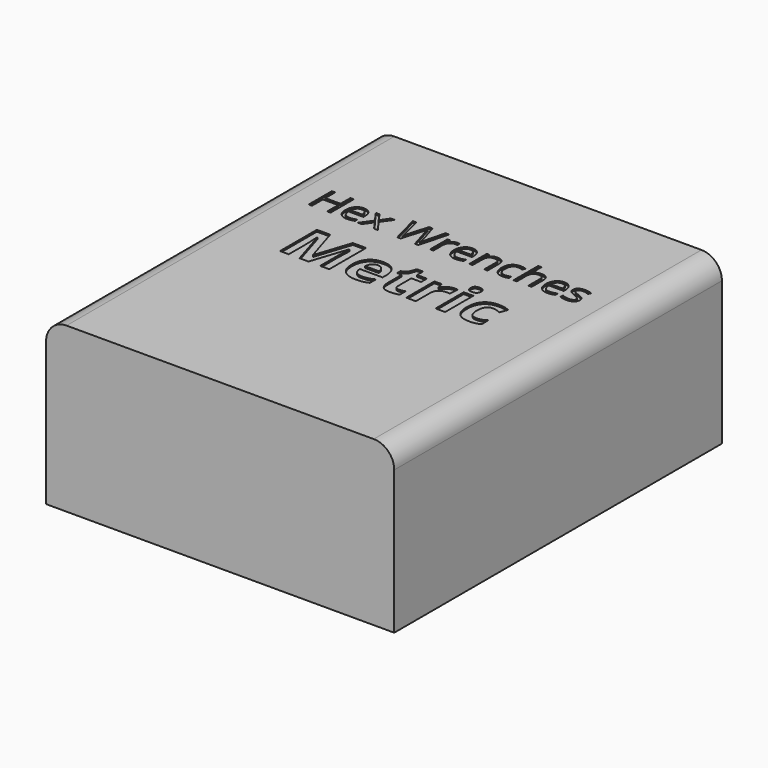
from build123d import *

# Parameters (mm, degrees)
F0_W           = 51.0000002086
F0_H           = 24.0000002086
F0_W_2         = 47
F0_H_2         = 20
F1_DEPTH       = 60
F2_R           = 3
F3_W           = 47
F3_H           = 20
F4_DEPTH       = 1
F5_TEXT_SIZE   = 5.9360942355
F5_TEXT_SIZE_2 = 9.4527740859
F6_DEPTH       = 0.25


# Not quite as in the source:
# - Text() gives the source's letters only with a copy of the font that has no kerning and outlines rounded to 1/6400 em; it was checked with that copy


with BuildPart() as f1:
    # F0 (on Front) → F1 (new body)
    with BuildSketch(Plane.XZ):
        Rectangle(F0_W, F0_H)
        Rectangle(F0_W_2, F0_H_2, mode=Mode.SUBTRACT)
    extrude(amount=F1_DEPTH)

    # F2
    f2_edges = [f1.edges().sort_by_distance(p)[0] for p in [
        (-25.5, -30, 12),
        (25.5, -30, 12),
    ]]
    fillet(f2_edges, radius=F2_R)

    # F3 (on face) → F4 (join)
    with BuildSketch(Plane.XZ.offset(60)):
        Rectangle(F3_W, F3_H)
    extrude(amount=-F4_DEPTH)

    # F5 (on face) → F6 (cut, symmetric)
    with BuildSketch(Plane.XY.offset(12.0000001043)):
        with Locations((-20.1936398028, -19.2833579477)):
            Text('Hex Wrenches', F5_TEXT_SIZE, font='Open Sans', text_align=(TextAlign.LEFT, TextAlign.BOTTOM))
        with Locations((-15.8186899498, -30.32877855)):
            Text('Metric', F5_TEXT_SIZE_2, font='Open Sans', font_style=FontStyle.BOLD, text_align=(TextAlign.LEFT, TextAlign.BOTTOM))
    extrude(amount=F6_DEPTH, both=True, mode=Mode.SUBTRACT)


solid = f1.part
